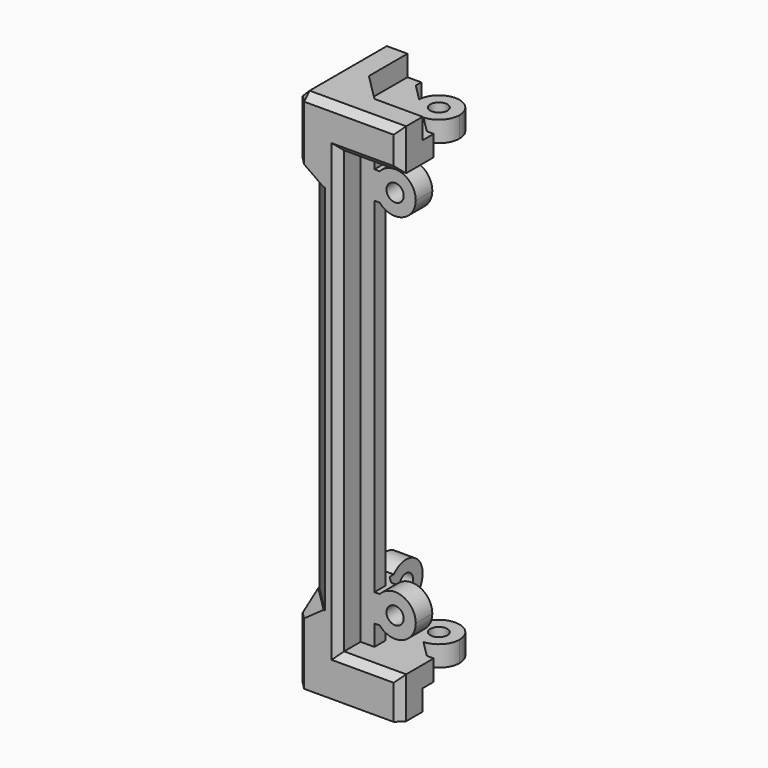
from build123d import *

# Parameters (mm, degrees)
F1_DEPTH  = 6
F2_W      = 2
F2_H      = 2
F3_DEPTH  = 5
F5_DEPTH  = 27
F7_DEPTH  = 3
F8_R      = 1.25
F9_DEPTH  = 3
F11_DEPTH = 4
F13_DEPTH = 3
F15_DEPTH = 3
F17_SIZE  = 0.99999
F18_SIZE  = 2


# Not quite as in the source:
# - a fillet or chamfer is up to 0.001 mm smaller than in the source, because OpenCascade refuses the exact size
# - a feature names something its author has since deleted; it is built from what else it names


with BuildPart() as f1:
    # F0 (on Top) → F1 (new body)
    with BuildSketch(Plane.XY):
        Polygon((-29.7051688433, 8.7922193985), (-30.7051688433, 8.7922193985), (-30.7051688433, -6.2077806015), (-15.7051688433, -6.2077806015), (-15.7051688433, -5.2077806015), (-15.7051688433, -0.2077806015), (-24.7051688433, -0.2077806015), (-24.7051688433, 8.7922193985), align=None)
    extrude(amount=F1_DEPTH)

    # F2 (on face) → F3 (join)
    with BuildSketch(Plane.XY.offset(6)):
        with Locations((-23.7051688433, -1.2077806015)):
            Rectangle(F2_W, F2_H)
        Polygon((-26.7051688433, -0.2077806015), (-30.7051688433, -0.2077806015), (-30.7051688433, -5.2077806015), (-29.7051688433, -6.2077806015), (-24.7051688433, -6.2077806015), (-24.7051688433, -2.2077806015), (-24.7051688433, -0.2077806015), align=None)
        with Locations((-25.7051688433, 0.7922193985)):
            Rectangle(F2_W, F2_H)
    extrude(amount=F3_DEPTH)

    # F4 (on face) → F5 (join)
    with BuildSketch(Plane.XY.offset(11)):
        Polygon((-26.7051688433, -6.2077806015), (-24.7051688433, -6.2077806015), (-24.7051688433, -2.2077806015), (-22.7051688433, -2.2077806015), (-22.7051688433, -0.2077806015), (-24.7051688433, -0.2077806015), (-24.7051688433, 1.7922193985), (-26.7051688433, 1.7922193985), (-26.7051688433, -0.2077806015), (-30.7051688433, -0.2077806015), (-30.7051688433, -2.2077806015), align=None)
    extrude(amount=F5_DEPTH)

    # F6 (on face) → F7 (join)
    with BuildSketch(Plane.XZ.offset(2.2077806015)):
        with BuildLine():
            ThreePointArc((-21.9412368208, 13), (-22.5076859202, 12.0704662693), (-22.7051688433, 11))
            ThreePointArc((-22.7051688433, 11), (-22.5076859202, 9.9295337307), (-21.9412368208, 9))
            ThreePointArc((-21.9412368208, 9), (-18.634702574, 8.1974829231), (-16.7051688433, 11))
            ThreePointArc((-16.7051688433, 11), (-18.634702574, 13.8025170769), (-21.9412368208, 13))
        make_face()
        with BuildLine():
            ThreePointArc((-18.4551688433, 11), (-19.7051688433, 9.75), (-20.9551688433, 11))
            ThreePointArc((-20.9551688433, 11), (-19.7051688433, 12.25), (-18.4551688433, 11))
        make_face(mode=Mode.SUBTRACT)
        with BuildLine():
            Line((-22.7051688433, 13), (-22.7051688433, 11))
            ThreePointArc((-22.7051688433, 11), (-22.5076859202, 12.0704662693), (-21.9412368208, 13))
            Line((-21.9412368208, 13), (-22.7051688433, 13))
        make_face()
        with BuildLine():
            Line((-22.7051688433, 11), (-22.7051688433, 9))
            Line((-22.7051688433, 9), (-21.9412368208, 9))
            ThreePointArc((-21.9412368208, 9), (-22.5076859202, 9.9295337307), (-22.7051688433, 11))
        make_face()
    extrude(amount=-F7_DEPTH)

    # F8 (on face) → F9 (join)
    with BuildSketch(Plane(origin=(-26.7051688433, 0, 0), x_dir=(0, -1, 0), z_dir=(-1, 0, 0))):
        with BuildLine():
            Line((-2.556151421, 9), (-1.7922193985, 9))
            Line((-1.7922193985, 9), (-1.7922193985, 11))
            ThreePointArc((-1.7922193985, 11), (-1.9897023217, 9.9295337307), (-2.556151421, 9))
        make_face()
        with BuildLine():
            ThreePointArc((-2.556151421, 13), (-1.9897023217, 12.0704662693), (-1.7922193985, 11))
            Line((-1.7922193985, 11), (-1.7922193985, 13))
            Line((-1.7922193985, 13), (-2.556151421, 13))
        make_face()
        with BuildLine():
            ThreePointArc((-2.556151421, 9), (-1.9897023217, 9.9295337307), (-1.7922193985, 11))
            ThreePointArc((-1.7922193985, 11), (-1.9897023217, 12.0704662693), (-2.556151421, 13))
            ThreePointArc((-2.556151421, 13), (-7.7922193985, 11), (-2.556151421, 9))
        make_face()
        with Locations((-4.7922193985, 11)):
            Circle(F8_R, mode=Mode.SUBTRACT)
    extrude(amount=-F9_DEPTH)

    # F10 (on face) → F11 (join)
    with BuildSketch(Plane.XY.offset(13)):
        Polygon((-22.7051688433, 0.7922193985), (-23.7051688433, 1.7922193985), (-24.7051688433, 1.7922193985), (-24.7051688433, -0.2077806015), (-22.7051688433, -0.2077806015), align=None)
    extrude(amount=-F11_DEPTH)

    # F12 (on face) → F13 (cut)
    with BuildSketch(Plane(origin=(0, 0, 0), x_dir=(1, 0, 0), z_dir=(0, 0, -1))):
        Polygon((-24.7051688433, -8.7922193985), (-24.7051688433, 0.2077806015), (-26.7051688433, -1.7922193985), (-26.7051688433, -8.7922193985), align=None)
        Polygon((-24.7051688433, 0.2077806015), (-15.7051688433, 0.2077806015), (-15.7051688433, 2.2077806015), (-22.7051688433, 2.2077806015), align=None)
    extrude(amount=-F13_DEPTH, mode=Mode.SUBTRACT)

    # F14 (on face) → F15 (join)
    with BuildSketch(Plane(origin=(0, 0, 3), x_dir=(1, 0, 0), z_dir=(0, 0, -1))):
        with BuildLine():
            Line((-16.7051688433, 0.2077806015), (-24.7051688433, 0.2077806015))
            Line((-24.7051688433, 0.2077806015), (-24.7051688433, -7.7922193985))
            Line((-24.7051688433, -7.7922193985), (-22.2863076734, -5.3733582286))
            ThreePointArc((-22.2863076734, -5.3733582286), (-21.4122756245, -3.0851126174), (-19.1240300132, -2.2110805685))
            Line((-19.1240300132, -2.2110805685), (-16.7051688433, 0.2077806015))
        make_face()
        with BuildLine():
            ThreePointArc((-19.1240300132, -2.2110805685), (-21.4122756245, -3.0851126174), (-22.2863076734, -5.3733582286))
            Line((-22.2863076734, -5.3733582286), (-20.7051688433, -3.7922193985))
            Line((-20.7051688433, -3.7922193985), (-19.1240300132, -2.2110805685))
        make_face()
        with BuildLine():
            Line((-20.7051688433, -3.7922193985), (-22.2863076734, -5.3733582286))
            ThreePointArc((-22.2863076734, -5.3733582286), (-19.2074603031, -8.2052708339), (-16.2909552809, -5.2064329609))
            ThreePointArc((-16.2909552809, -5.2064329609), (-17.1114168202, -3.1449742302), (-19.1240300132, -2.2110805685))
            Line((-19.1240300132, -2.2110805685), (-20.7051688433, -3.7922193985))
        make_face()
        with BuildLine():
            ThreePointArc((-18.0409552809, -5.2064329609), (-19.7693095714, -6.3612823766), (-20.1748387574, -4.3225494844))
            ThreePointArc((-20.1748387574, -4.3225494844), (-18.8126009904, -4.0515835453), (-18.0409552809, -5.2064329609))
        make_face(mode=Mode.SUBTRACT)
    extrude(amount=-F15_DEPTH)

    # F16: F1 across face


with BuildPart() as f1_1:
    add(f1.part)
    add(f1.part.mirror(Plane(origin=(-26.6681318062, -2.1707435644, 38), x_dir=(1, 0, 0), z_dir=(0, 0, 1))))

    # F17 (size 1 in the source; OpenCascade refuses exactly that, so slightly less here)
    f17_edges = [f1_1.edges().sort_by_distance(p)[0] for p in [
        (-24.705169, -6.207781, 38),
        (-20.205169, -6.207781, 6),
        (-30.705169, 4.292219, 6),
        (-30.705169, -0.207781, 38),
        (-30.705169, 4.292219, 70),
        (-20.205169, -6.207781, 70),
        (-15.705169, -6.207781, 73),
        (-30.705169, 8.792219, 73),
        (-23.205169, -6.207781, 76),
        (-30.705169, -6.207781, 73),
        (-30.705169, 1.292219, 76),
        (-30.705169, 8.792219, 3),
        (-30.705169, -6.207781, 3),
        (-15.705169, -6.207781, 3),
    ]]
    chamfer(f17_edges, length=F17_SIZE)

    # F18
    f18_edges = [f1_1.edges().sort_by_distance(p)[0] for p in [
        (-30.205169, -5.707781, 11),
        (-30.205169, -5.707781, 65),
    ]]
    chamfer(f18_edges, length=F18_SIZE)


solid = f1_1.part
